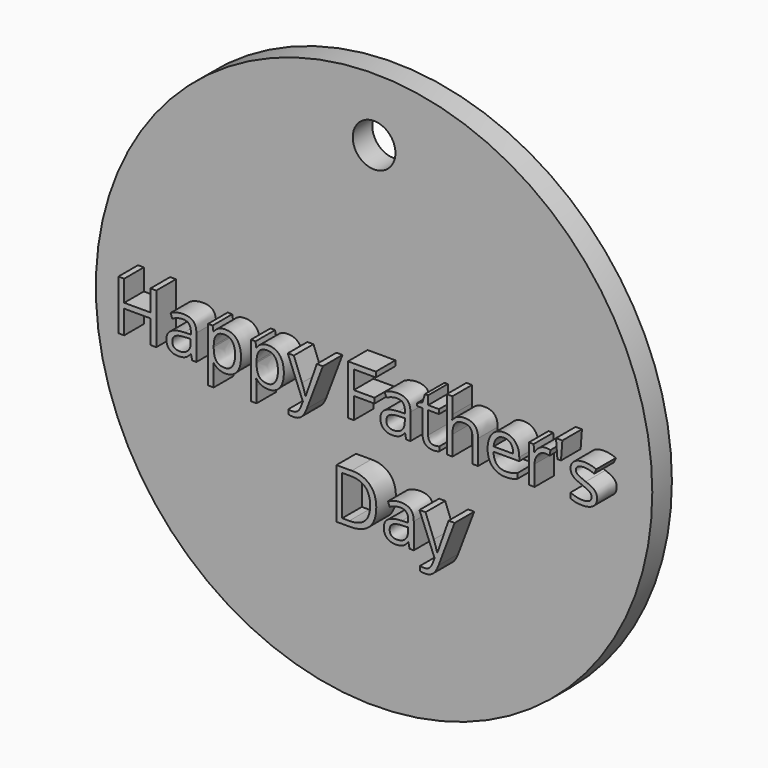
from build123d import *

# Parameters (mm, degrees)
F0_R         = 36.053226602
F1_DEPTH     = 3.175
F2_TEXT_SIZE = 9.0601034421
F3_DEPTH     = 3.175
F4_R         = 2.7657898724
F5_DEPTH     = 12.7


# Not quite as in the source:
# - Text() gives the source's letters only with a copy of the font that has no kerning and outlines rounded to 1/6400 em; it was checked with that copy


with BuildPart() as f1:
    # F0 (on Front) → F1 (new body)
    with BuildSketch(Plane.XZ):
        Circle(F0_R)
    extrude(amount=F1_DEPTH)

    # F2 (on face) → F3 (join)
    with BuildSketch(Plane.XZ.offset(3.175)):
        with Locations((-31.4757385742, -2.2221663201)):
            Text("Happy Father's", F2_TEXT_SIZE, font='Open Sans', text_align=(TextAlign.LEFT, TextAlign.BOTTOM))
        with Locations((-3.2252035287, -14.5439070014)):
            Text('Day', F2_TEXT_SIZE, font='Open Sans', text_align=(TextAlign.LEFT, TextAlign.BOTTOM))
    extrude(amount=F3_DEPTH)

    # F4 (on face) → F5 (cut, symmetric)
    with BuildSketch(Plane.XZ.offset(3.175)):
        with Locations((0, 27.8866812587)):
            Circle(F4_R)
    extrude(amount=F5_DEPTH, both=True, mode=Mode.SUBTRACT)


solid = f1.part
